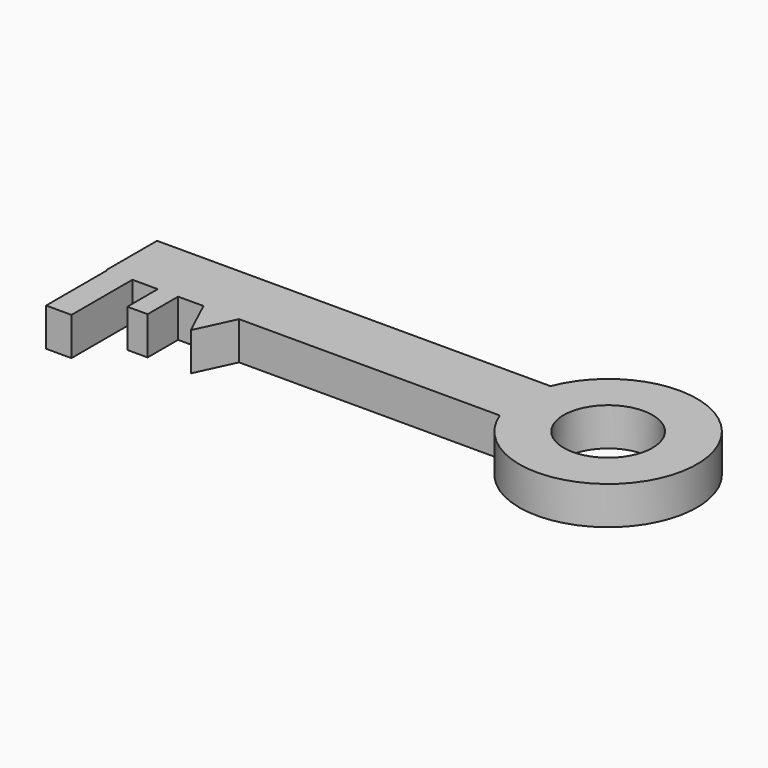
from build123d import *

# Parameters (mm, degrees)
F0_R     = 17.5
F0_W     = 10
F0_H     = 30
F0_W_2   = 8
F0_H_2   = 15
F1_DEPTH = 15


# Not quite as in the source:
# - a feature of the source that left no trace in its solid (it failed there, or was rolled back) is left out


with BuildPart() as f1:
    # F0 (on Top) → F1 (new body)
    with BuildSketch(Plane.XY):
        with BuildLine():
            Line((60.2198065221, 40), (-94.7801934779, 40))
            Line((-94.7801934779, 40), (-94.7801934779, 15))
            Line((-94.7801934779, 15), (-94.4899649718, 15))
            Line((-94.4899649718, 15), (-84.4899649718, 15))
            Line((-84.4899649718, 15), (-74.4899649718, 15))
            Line((-74.4899649718, 15), (-66.4899649718, 15))
            Line((-66.4899649718, 15), (-56.4899649718, 15))
            Line((-56.4899649718, 15), (-42.4899649718, 15))
            Line((-42.4899649718, 15), (60.2198065221, 15))
            ThreePointArc((60.2198065221, 15), (127.9115485987, 27.5), (60.2198065221, 40))
        make_face()
        with Locations((92.9115485987, 27.5)):
            Circle(F0_R, mode=Mode.SUBTRACT)
        with Locations((-89.4899649718, 0)):
            Rectangle(F0_W, F0_H)
        with Locations((-70.4899649718, 7.5)):
            Rectangle(F0_W_2, F0_H_2)
        Polygon((-49.4899649718, 0), (-42.4899649718, 15), (-56.4899649718, 15), align=None)
    extrude(amount=F1_DEPTH)


solid = f1.part
